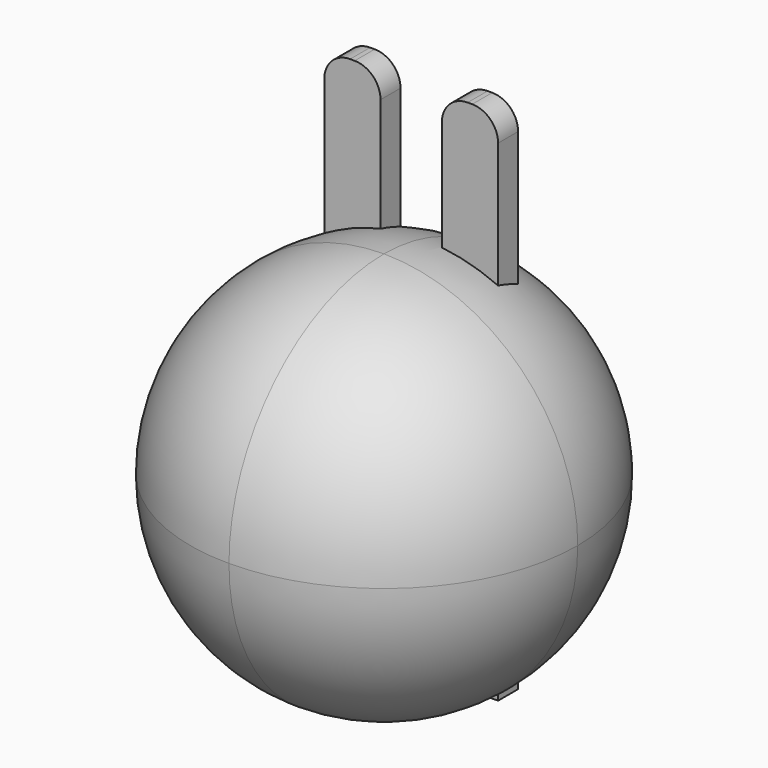
from build123d import *

# Parameters (mm, degrees)
F0_W     = 30
F0_H     = 30
F1_DEPTH = 30
F2_R     = 14.99999
F3_W     = 4.3548396789
F3_H     = 1.9354838878
F4_DEPTH = 40
F5_R     = 2


# Not quite as in the source:
# - a fillet or chamfer is up to 0.001 mm smaller than in the source, because OpenCascade refuses the exact size
# - the program builds the solid bodies; features that only make, move or delete a surface that nothing else refers to are left out


with BuildPart() as f1:
    # F0 (on Top) → F1 (new body)
    with BuildSketch(Plane.XY):
        Rectangle(F0_W, F0_H)
    extrude(amount=F1_DEPTH)

    # F2 (radius 15 in the source; OpenCascade refuses exactly that, so slightly less here)
    f2_edges = [f1.edges().sort_by_distance(p)[0] for p in [
        (-15, -15, 15),
        (-15, 0, 30),
        (0, -15, 30),
        (0, 15, 30),
        (15, 0, 30),
        (15, 15, 15),
        (-15, 15, 15),
        (0, 15, 0),
        (-15, 0, 0),
        (0, -15, 0),
        (15, 0, 0),
        (15, -15, 15),
    ]]
    fillet(f2_edges, radius=F2_R)

    # F3 (on Top) → F4 (join)
    with BuildSketch(Plane.XY):
        with Locations((3.7499994505, 4.5967744663)):
            Rectangle(F3_W, F3_H)
        with Locations((-5.3500005495, 4.5967744663)):
            Rectangle(F3_W, F3_H)
    extrude(amount=F4_DEPTH)

    # F5
    f5_edges = [f1.edges().sort_by_distance(p)[0] for p in [
        (5.927419, 4.596774, 40),
        (-3.172581, 4.596774, 40),
        (1.57258, 4.596774, 40),
        (-7.52742, 4.596774, 40),
    ]]
    fillet(f5_edges, radius=F5_R)


solid = f1.part
